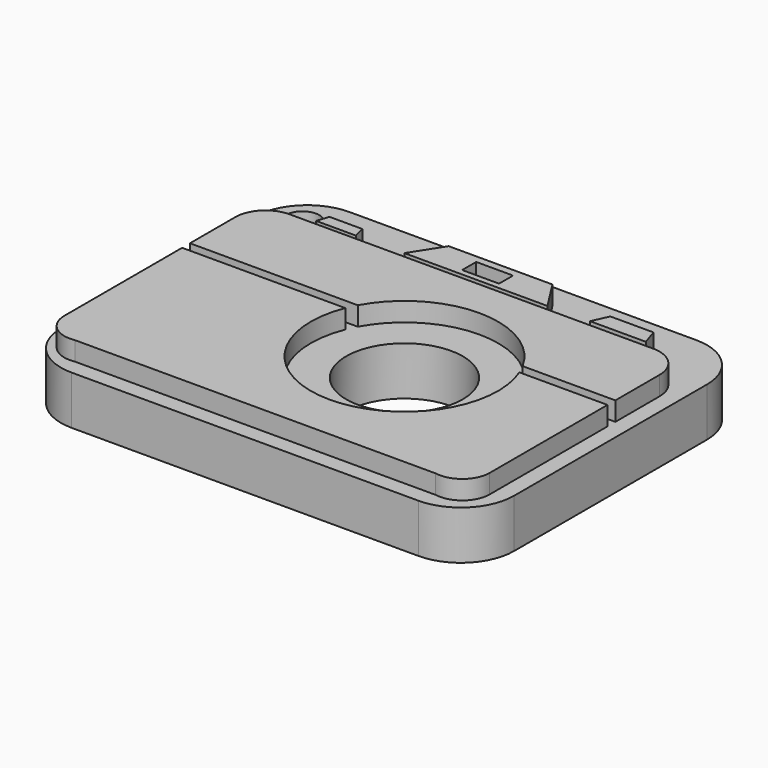
from build123d import *

# Parameters (mm, degrees)
F1_DEPTH = 6.35
F0_R     = 5.481735544
F0_R_2   = 1.5875
F2_DEPTH = 4.572


# Not quite as in the source:
# - ends of sketch curves that miss each other by under 0.0002 mm in the source are joined


with BuildPart() as f1:
    # F0 (on Top) → F1 (new body)
    with BuildSketch(Plane.XY):
        with BuildLine():
            ThreePointArc((-19.4521045311, 6.5193053193), (-21.5031469057, 5.6399822857), (-22.2801735623, 3.5480421826))
            Line((-22.2801735623, 3.5480421826), (-22.2801735623, -1.6389441203))
            Line((-22.2801735623, -1.6389441203), (-6.5127791505, -1.6389441203))
            ThreePointArc((-6.5127791505, -1.6389441203), (1.2310059125, 2.972369205), (8.9747909756, -1.6389441203))
            Line((8.9747909756, -1.6389441203), (17.6922247706, -1.6389441203))
            Line((17.6922247706, -1.6389441203), (17.6922247706, 3.5480415082))
            ThreePointArc((17.6922247706, 3.5480415082), (16.8726231039, 5.5978906933), (14.8656907599, 6.5175923519))
            Line((14.8656907599, 6.5175923519), (-19.4521045311, 6.5193053193))
        make_face()
    extrude(amount=F1_DEPTH)


with BuildPart() as f1b:
    # F0 (on Top) → F1, piece 2 (new body)
    with BuildSketch(Plane.XY):
        with BuildLine():
            Line((-22.2801735623, -2.5610408197), (-22.2801735623, -16.3933522999))
            ThreePointArc((-22.2801735623, -16.3933522999), (-21.3530783029, -18.375721012), (-19.2373136057, -18.9350340515))
            Line((-19.2373136057, -18.9350340515), (-2.2932069786, -18.9350340515))
            Line((-2.2932069786, -18.9350340515), (14.6508998345, -18.9350340515))
            ThreePointArc((14.6508998345, -18.9350340515), (16.7658482764, -18.3739688541), (17.6922247706, -16.3916400069))
            Line((17.6922247706, -16.3916400069), (17.6922247706, -2.5610408197))
            Line((17.6922247706, -2.5610408197), (9.4074936158, -2.5610408197))
            ThreePointArc((9.4074936158, -2.5610408197), (1.2310059125, -14.6430934532), (-6.9454817907, -2.5610408197))
            Line((-6.9454817907, -2.5610408197), (-22.2801735623, -2.5610408197))
        make_face()
    extrude(amount=F1_DEPTH)


with BuildPart() as f1c:
    # F0 (on Top) → F1, piece 3 (new body)
    with BuildSketch(Plane.XY):
        Polygon((2.5806244571, 9.8610082641), (-2.2932067925, 9.8610082641), (-7.1670380421, 9.8610082641), (-9.0154232457, 6.9678835571), (-2.2932067925, 6.9678835571), (4.4290096607, 6.9678835571), align=None)
        Polygon((-4.0268255398, 9.1632921249), (-2.2932067925, 9.1632921249), (-0.5595880453, 9.1632921249), (-0.5595880453, 7.516568061), (-2.2932067925, 7.516568061), (-4.0268255398, 7.516568061), align=None, mode=Mode.SUBTRACT)
    extrude(amount=F1_DEPTH)


with BuildPart() as f1d:
    # F0 (on Top) → F1, piece 4 (new body)
    with BuildSketch(Plane.XY):
        Polygon((-13.8089191169, 8.0332169309), (-16.9094987214, 8.0332169309), (-17.2707308084, 6.919416599), (-16.5636505928, 6.919416599), (-14.1506345941, 6.919416599), (-13.5379955173, 6.919416599), align=None)
    extrude(amount=F1_DEPTH)


with BuildPart() as f1e:
    # F0 (on Top) → F1, piece 5 (new body)
    with BuildSketch(Plane.XY):
        Polygon((9.0685896575, 8.5486769676), (8.3859022707, 7.0315953344), (9.4382846728, 7.0315953344), (12.5052956864, 7.0315953344), (13.6198326945, 7.0315953344), (13.1267812103, 8.5486769676), align=None)
    extrude(amount=F1_DEPTH)


with BuildPart() as f2:
    # F0 (on Top) → F2 (new body)
    with BuildSketch(Plane.XY):
        with BuildLine():
            Line((14.2269962281, 12.2182751074), (-18.3607199043, 12.2182751074))
            ThreePointArc((-18.3607199043, 12.2182751074), (-21.8962538102, 10.7538090134), (-23.3607199043, 7.2182751074))
            Line((-23.3607199043, 7.2182751074), (-23.3607199043, -15.4466097057))
            ThreePointArc((-23.3607199043, -15.4466097057), (-21.8962538102, -18.9821436116), (-18.3607199043, -20.4466097057))
            Line((-18.3607199043, -20.4466097057), (14.2269962281, -20.4466097057))
            ThreePointArc((14.2269962281, -20.4466097057), (17.762530134, -18.9821436116), (19.2269962281, -15.4466097057))
            Line((19.2269962281, -15.4466097057), (19.2269962281, 7.2182751074))
            ThreePointArc((19.2269962281, 7.2182751074), (17.762530134, 10.7538090134), (14.2269962281, 12.2182751074))
        make_face()
        with BuildLine():
            ThreePointArc((-19.2373136057, -18.9350340515), (-21.3530783029, -18.375721012), (-22.2801735623, -16.3933522999))
            Line((-22.2801735623, -16.3933522999), (-22.2801735623, -2.5610408197))
            Line((-22.2801735623, -2.5610408197), (-6.9454817907, -2.5610408197))
            ThreePointArc((-6.9454817907, -2.5610408197), (1.2310059125, -14.6430934532), (9.4074936158, -2.5610408197))
            Line((9.4074936158, -2.5610408197), (17.6922247706, -2.5610408197))
            Line((17.6922247706, -2.5610408197), (17.6922247706, -16.3916400069))
            ThreePointArc((17.6922247706, -16.3916400069), (16.7658482764, -18.3739688541), (14.6508998345, -18.9350340515))
            Line((14.6508998345, -18.9350340515), (-2.2932067925, -18.9350340515))
            Line((-2.2932067925, -18.9350340515), (-19.2373136057, -18.9350340515))
        make_face(mode=Mode.SUBTRACT)
        with Locations((1.2310059125, -5.8353621241)):
            Circle(F0_R, mode=Mode.SUBTRACT)
        with BuildLine():
            Line((-22.2801735623, -1.6389441203), (-22.2801735623, 3.5480421826))
            ThreePointArc((-22.2801735623, 3.5480421826), (-21.5031469057, 5.6399822857), (-19.4521045311, 6.5193053193))
            Line((-19.4521045311, 6.5193053193), (14.8656907599, 6.5175923519))
            ThreePointArc((14.8656907599, 6.5175923519), (16.8726231039, 5.5978906933), (17.6922247706, 3.5480415082))
            Line((17.6922247706, 3.5480415082), (17.6922247706, -1.6389441203))
            Line((17.6922247706, -1.6389441203), (8.9747909756, -1.6389441203))
            ThreePointArc((8.9747909756, -1.6389441203), (1.2310059125, 2.972369205), (-6.5127791505, -1.6389441203))
            Line((-6.5127791505, -1.6389441203), (-22.2801735623, -1.6389441203))
        make_face(mode=Mode.SUBTRACT)
        Polygon((-17.2707308084, 6.919416599), (-16.9094987214, 8.0332169309), (-13.8089191169, 8.0332169309), (-13.5379955173, 6.919416599), (-14.1506345941, 6.919416599), (-16.5636505928, 6.919416599), align=None, mode=Mode.SUBTRACT)
        with Locations((-20.1489608735, 8.9084757492)):
            Circle(F0_R_2, mode=Mode.SUBTRACT)
        Polygon((-7.1670380421, 9.8610082641), (-2.2932067925, 9.8610082641), (2.5806244571, 9.8610082641), (4.4290096607, 6.9678835571), (-2.2932067925, 6.9678835571), (-9.0154232457, 6.9678835571), align=None, mode=Mode.SUBTRACT)
        Polygon((9.4382846728, 7.0315953344), (8.3859022707, 7.0315953344), (9.0685896575, 8.5486769676), (13.1267812103, 8.5486769676), (13.6198326945, 7.0315953344), (12.5052956864, 7.0315953344), align=None, mode=Mode.SUBTRACT)
    extrude(amount=F2_DEPTH)


solid = Compound([f1.part, f1b.part, f1c.part, f1d.part, f1e.part, f2.part])
